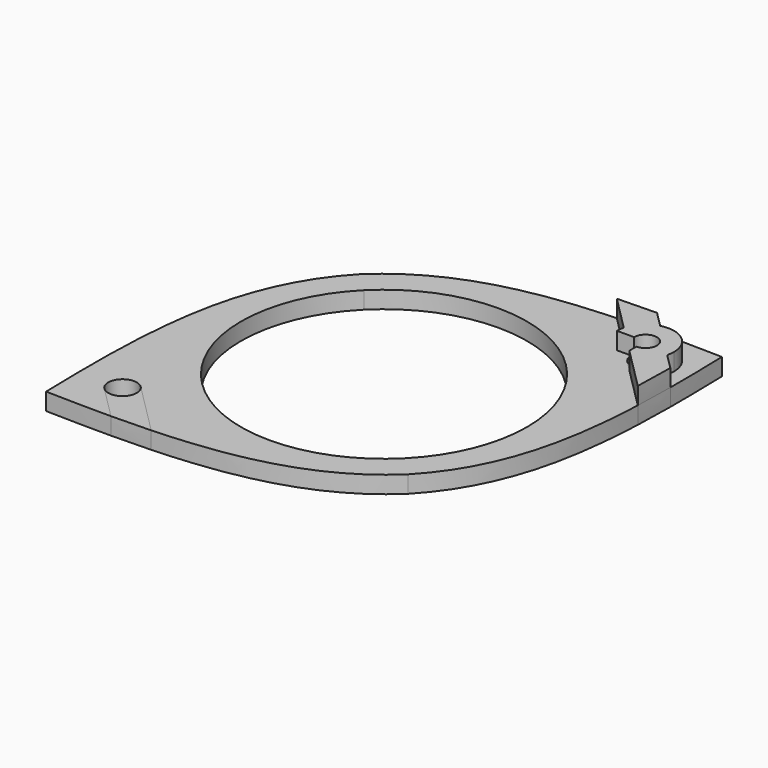
from build123d import *

# Parameters (mm, degrees)
F1_DEPTH = 3
F2_DEPTH = 3
F4_DEPTH = 3


with BuildPart() as f1:
    # F0 (on Top) → F1 (new body)
    with BuildSketch(Plane.XY):
        with BuildLine():
            Line((-17.6776695297, 17.6776695297), (-21.0540489196, 21.0540489196))
            add(Edge.make_bspline(
                [(-21.0540489196, 21.0540489196), (-32.6172978292, 8.9064244237), (-33.4403195997, -9.1381745127), (-32.823822752, -32.823822752)],
                knots=[5.6905599108, 5.6905599108, 5.6905599108, 5.6905599108, 59.653525178, 59.653525178, 59.653525178, 59.653525178], degree=3))
            add(Edge.make_bspline(
                [(-21.3653856494, -32.9685513557), (-25.0248508067, -32.9903335411), (-28.8447343113, -32.9273916076), (-32.823822752, -32.823822752)],
                knots=[50.5879758987, 50.5879758987, 50.5879758987, 50.5879758987, 59.653525178, 59.653525178, 59.653525178, 59.653525178], degree=3))
            Line((-21.3653856494, -32.9685513557), (-27.1669685025, -27.1669685025))
            ThreePointArc((-27.1669685025, -27.1669685025), (-27.1669685025, -23.6314345966), (-23.6314345966, -23.6314345966))
            Line((-23.6314345966, -23.6314345966), (-14.4553227676, -32.8075464256))
            add(Edge.make_bspline(
                [(21.0540489196, -21.0540489196), (12.269278567, -29.4162176905), (0.400558033, -32.1615526479), (-14.4553227676, -32.8075464256)],
                knots=[5.6905599108, 5.6905599108, 5.6905599108, 5.6905599108, 44.7148364329, 44.7148364329, 44.7148364329, 44.7148364329], degree=3))
            add(Edge.make_bspline(
                [(21.0540489196, -21.0540489196), (29.4162176905, -12.269278567), (32.1615526479, -0.400558033), (32.8075464256, 14.4553227676)],
                knots=[5.6905599108, 5.6905599108, 5.6905599108, 5.6905599108, 44.7148364329, 44.7148364329, 44.7148364329, 44.7148364329], degree=3))
            Line((32.8075464256, 14.4553227676), (23.6314345966, 23.6314345966))
            Line((23.6314345966, 23.6314345966), (17.6776695297, 17.6776695297))
            ThreePointArc((17.6776695297, 17.6776695297), (25, 0), (17.6776695297, -17.6776695297))
            ThreePointArc((17.6776695297, -17.6776695297), (0, -25), (-17.6776695297, -17.6776695297))
            ThreePointArc((-17.6776695297, -17.6776695297), (-25, 0), (-17.6776695297, 17.6776695297))
        make_face()
        with BuildLine():
            add(Edge.make_bspline(
                [(-21.0540489196, 21.0540489196), (-8.9064244237, 32.6172978292), (9.1381745127, 33.4403195997), (32.823822752, 32.823822752)],
                knots=[5.6905599108, 5.6905599108, 5.6905599108, 5.6905599108, 59.653525178, 59.653525178, 59.653525178, 59.653525178], degree=3))
            Line((-21.0540489196, 21.0540489196), (-17.6776695297, 17.6776695297))
            ThreePointArc((-17.6776695297, 17.6776695297), (0, 25), (17.6776695297, 17.6776695297))
            Line((17.6776695297, 17.6776695297), (23.6314345966, 23.6314345966))
            ThreePointArc((23.6314345966, 23.6314345966), (23.6314345966, 27.1669685025), (27.1669685025, 27.1669685025))
            Line((27.1669685025, 27.1669685025), (32.823822752, 32.823822752))
        make_face()
        with BuildLine():
            add(Edge.make_bspline(
                [(32.9685513557, 21.3653856494), (32.9903335411, 25.0248508067), (32.9273916076, 28.8447343113), (32.823822752, 32.823822752)],
                knots=[50.5879758987, 50.5879758987, 50.5879758987, 50.5879758987, 59.653525178, 59.653525178, 59.653525178, 59.653525178], degree=3))
            Line((32.823822752, 32.823822752), (27.1669685025, 27.1669685025))
            Line((27.1669685025, 27.1669685025), (32.9685513557, 21.3653856494))
        make_face()
    extrude(amount=F1_DEPTH)


with BuildPart() as f2:
    # F0 (on Top) → F2 (new body)
    with BuildSketch(Plane.XY):
        with BuildLine():
            Line((32.9685513557, 21.3653856494), (27.1669685025, 27.1669685025))
            ThreePointArc((27.1669685025, 27.1669685025), (27.7089003809, 26.3559101305), (27.8992015496, 25.3992015496))
            ThreePointArc((27.8992015496, 25.3992015496), (26.3559101305, 23.0895027183), (23.6314345966, 23.6314345966))
            Line((23.6314345966, 23.6314345966), (32.8075464256, 14.4553227676))
            add(Edge.make_bspline(
                [(32.8075464256, 14.4553227676), (32.9047682549, 16.6911274411), (32.9544397107, 18.9945917154), (32.9685513557, 21.3653856494)],
                knots=[44.7148364329, 44.7148364329, 44.7148364329, 44.7148364329, 50.5879758987, 50.5879758987, 50.5879758987, 50.5879758987], degree=3))
        make_face()
    extrude(amount=F2_DEPTH)


with BuildPart() as f2b:
    # F0 (on Top) → F2, piece 2 (new body)
    with BuildSketch(Plane.XY):
        with BuildLine():
            Line((-27.1669685025, -27.1669685025), (-21.3653856494, -32.9685513557))
            add(Edge.make_bspline(
                [(-14.4553227676, -32.8075464256), (-16.6911274411, -32.9047682549), (-18.9945917154, -32.9544397107), (-21.3653856494, -32.9685513557)],
                knots=[44.7148364329, 44.7148364329, 44.7148364329, 44.7148364329, 50.5879758987, 50.5879758987, 50.5879758987, 50.5879758987], degree=3))
            Line((-14.4553227676, -32.8075464256), (-23.6314345966, -23.6314345966))
            ThreePointArc((-23.6314345966, -23.6314345966), (-23.0895027183, -24.4424929687), (-22.8992015496, -25.3992015496))
            ThreePointArc((-22.8992015496, -25.3992015496), (-24.4424929687, -27.7089003809), (-27.1669685025, -27.1669685025))
        make_face()
    extrude(amount=F2_DEPTH)


with BuildPart() as f4:
    # F3 (on face) → F4 (new body)
    with BuildSketch(Plane.XY.offset(3)):
        with BuildLine():
            ThreePointArc((20.5695724181, 26.6932967751), (20.4419772427, 26.0518325107), (20.3992015496, 25.3992015496))
            Line((20.3992015496, 25.3992015496), (21.8636676436, 25.3992015496))
            Line((21.8636676436, 25.3992015496), (20.5695724181, 26.6932967751))
        make_face()
        with BuildLine():
            Line((25.3992015496, 21.8636676436), (26.6932967751, 20.5695724181))
            ThreePointArc((26.6932967751, 20.5695724181), (28.9347354555, 21.8636676436), (30.228830681, 24.1051063241))
            Line((30.228830681, 24.1051063241), (27.1669685025, 27.1669685025))
            ThreePointArc((27.1669685025, 27.1669685025), (24.4424929687, 27.7089003809), (22.8992015496, 25.3992015496))
            Line((22.8992015496, 25.3992015496), (23.3992015496, 25.3992015496))
            ThreePointArc((23.3992015496, 25.3992015496), (25.3992015496, 27.3992015496), (27.3992015496, 25.3992015496))
            ThreePointArc((27.3992015496, 25.3992015496), (26.8134151119, 23.9849879872), (25.3992015496, 23.3992015496))
            Line((25.3992015496, 23.3992015496), (25.3992015496, 21.8636676436))
        make_face()
        with BuildLine():
            ThreePointArc((30.228830681, 24.1051063241), (28.9347354555, 21.8636676436), (26.6932967751, 20.5695724181))
            Line((26.6932967751, 20.5695724181), (32.8075464256, 14.4553227676))
            add(Edge.make_bspline(
                [(32.8075464256, 14.4553227676), (32.9047682549, 16.6911274411), (32.9544397107, 18.9945917154), (32.9685513557, 21.3653856493)],
                knots=[0.7495757593, 0.7495757593, 0.7495757593, 0.7495757593, 0.8480299487, 0.8480299487, 0.8480299487, 0.8480299487], degree=3))
            Line((32.9685513557, 21.3653856494), (30.228830681, 24.1051063241))
        make_face()
        with BuildLine():
            Line((14.4553227676, 32.8075464256), (20.5695724181, 26.6932967751))
            ThreePointArc((20.5695724181, 26.6932967751), (21.8636676436, 28.9347354555), (24.1051063241, 30.228830681))
            Line((24.1051063241, 30.228830681), (21.3653856494, 32.9685513557))
            add(Edge.make_bspline(
                [(14.4553227676, 32.8075464256), (16.6911274411, 32.9047682549), (18.9945917154, 32.9544397107), (21.3653856493, 32.9685513557)],
                knots=[0.7495757593, 0.7495757593, 0.7495757593, 0.7495757593, 0.8480299487, 0.8480299487, 0.8480299487, 0.8480299487], degree=3))
        make_face()
        with BuildLine():
            ThreePointArc((24.1051063241, 30.228830681), (21.8636676436, 28.9347354555), (20.5695724181, 26.6932967751))
            Line((20.5695724181, 26.6932967751), (21.8636676436, 25.3992015496))
            Line((21.8636676436, 25.3992015496), (22.8992015496, 25.3992015496))
            ThreePointArc((22.8992015496, 25.3992015496), (24.4424929687, 27.7089003809), (27.1669685025, 27.1669685025))
            Line((27.1669685025, 27.1669685025), (24.1051063241, 30.228830681))
        make_face()
        with BuildLine():
            ThreePointArc((30.3992015496, 25.3992015496), (28.4430086946, 29.365968251), (24.1051063241, 30.228830681))
            Line((24.1051063241, 30.228830681), (27.1669685025, 27.1669685025))
            Line((27.1669685025, 27.1669685025), (30.228830681, 24.1051063241))
            ThreePointArc((30.228830681, 24.1051063241), (30.3564258564, 24.7465705885), (30.3992015496, 25.3992015496))
        make_face()
    extrude(amount=F4_DEPTH)


solid = Compound([f1.part, f2.part, f2b.part, f4.part])
